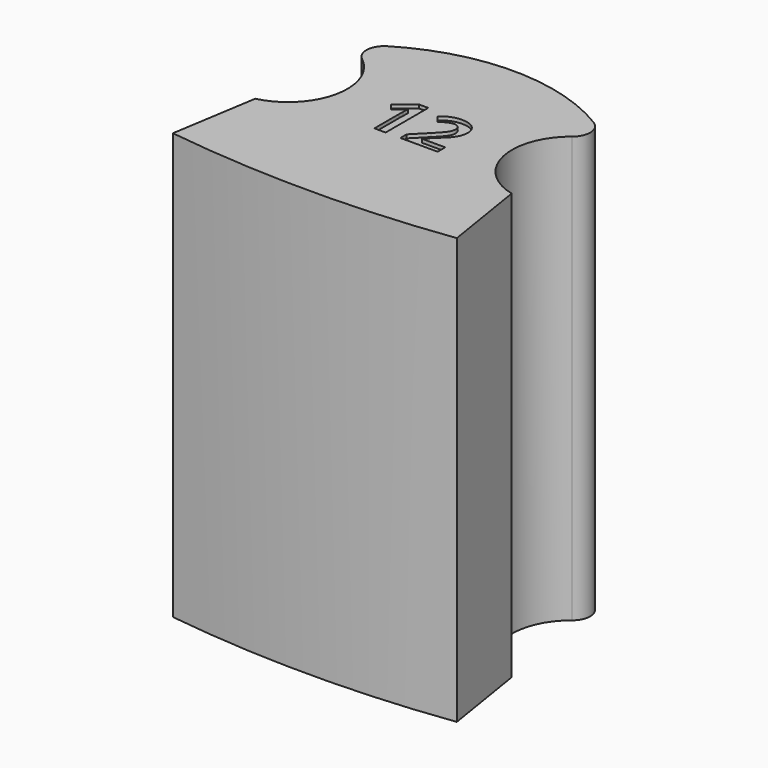
from build123d import *

# Parameters (mm, degrees)
F1_DEPTH     = 120
F2_TEXT_SIZE = 21.0426799539
F3_DEPTH     = 1


# Not quite as in the source:
# - Text() gives the source's letters only with a copy of the font that has no kerning and outlines rounded to 1/6400 em; it was checked with that copy


with BuildPart() as f1:
    # F0 (on Top) → F1 (new body)
    with BuildSketch(Plane.XY):
        with BuildLine():
            Line((3.8687128108, 24.1569802165), (0, 0))
            ThreePointArc((0, 0), (40, -2.6430687706), (80, 0))
            Line((80, 0), (76.1312871892, 24.1569802165))
            ThreePointArc((76.1312871892, 24.1569802165), (63.5975554576, 36.8458138953), (69.5972800683, 53.6417728094))
            ThreePointArc((69.5972800683, 53.6417728094), (71.4969098635, 57.8715436357), (69.1043731597, 61.843359684))
            ThreePointArc((69.1043731597, 61.843359684), (40, 70), (10.8956268403, 61.843359684))
            ThreePointArc((10.8956268403, 61.843359684), (8.5030901365, 57.8715436357), (10.4027199317, 53.6417728094))
            ThreePointArc((10.4027199317, 53.6417728094), (16.4024445424, 36.8458138953), (3.8687128108, 24.1569802165))
        make_face()
    extrude(amount=F1_DEPTH)

    # F2 (on face) → F3 (cut)
    with BuildSketch(Plane.XY.offset(120)):
        with Locations((27.6407134458, 29.5085348189)):
            Text('12', F2_TEXT_SIZE, font='Open Sans', font_style=FontStyle.BOLD, text_align=(TextAlign.LEFT, TextAlign.BOTTOM))
    extrude(amount=-F3_DEPTH, mode=Mode.SUBTRACT)


solid = f1.part
